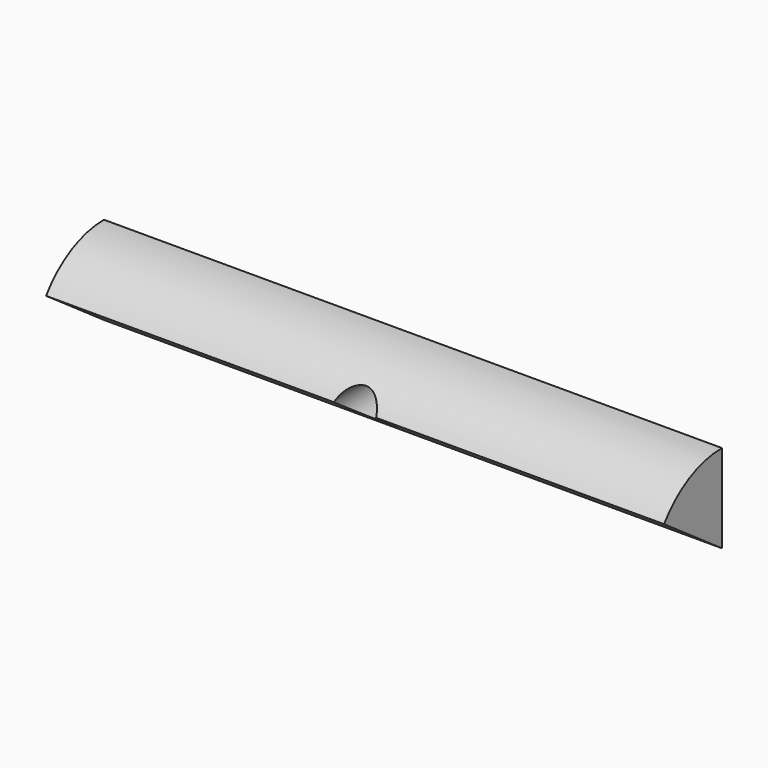
from build123d import *

# Parameters (mm, degrees)
F0_W     = 177.8
F0_H     = 25.4
F1_ANGLE = 55
F3_DEPTH = 20.8074619249
F5_R     = 6.35
F6_DEPTH = 16.51


with BuildPart() as f1:
    # F0 (on Front) → F1 (revolve)
    with BuildSketch(Plane.XZ):
        with Locations((88.9, 12.7)):
            Rectangle(F0_W, F0_H)
    revolve(axis=Axis((88.9, 0, 0), (1, 0, 0)), revolution_arc=F1_ANGLE)

    # F2 (on Front) → F3 (cut, through all)
    with BuildSketch(Plane.XZ):
        with BuildLine():
            ThreePointArc((88.9, 8.89), (91.5940768363, 10.0059231637), (92.71, 12.7))
            ThreePointArc((92.71, 12.7), (86.2059231637, 15.3940768363), (88.9, 8.89))
        make_face()
    extrude(amount=F3_DEPTH, mode=Mode.SUBTRACT)

    # F5 (on plane+point) → F6 (cut)
    with BuildSketch(Plane.XZ.offset(20.8064619249)):
        with Locations((88.9, 12.7)):
            Circle(F5_R)
    extrude(amount=-F6_DEPTH, mode=Mode.SUBTRACT)


solid = f1.part
